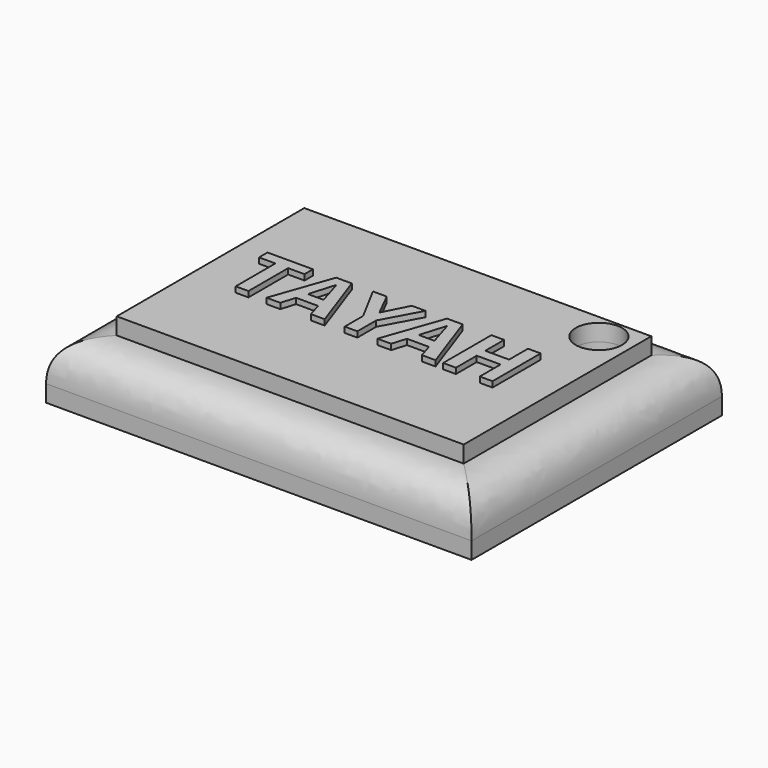
from build123d import *

# Parameters (mm, degrees)
F0_W         = 75.8890584111
F0_H         = 55.81606552
F1_DEPTH     = 10
F2_T1_DEPTH  = 110.8890584111
F2_T3_DEPTH  = 90.81606552
F3_DEPTH     = 3
F4_TEXT_SIZE = 15.0474936518
F6_DEPTH     = 1
F5_R         = 4.1296753225
F7_DEPTH     = 29.6


# Not quite as in the source:
# - a fillet or chamfer that OpenCascade refuses, or shapes differently, is made with other operations: its cross-section is extruded or revolved along the edge and cut away or added
# - Text() gives the source's letters only with a copy of the font that has no kerning and outlines rounded to 1/6400 em; it was checked with that copy


with BuildPart() as f1:
    # F0 (on Top) → F1 (new body)
    with BuildSketch(Plane.XY):
        with Locations((-37.9445292056, 27.90803276)):
            Rectangle(F0_W, F0_H)
    extrude(amount=F1_DEPTH)

    # F2: fillet of radius 7 on 4 edges, made by hand

    # F2_s2 → F2_t1 (cut)
    with BuildSketch(Plane.YZ.offset(-93.3890584111)):
        with BuildLine():
            add(Edge.make_bspline(
                [(0, 3), (0, 10), (7, 10)],
                knots=[0, 0, 0, 1, 1, 1], degree=2, weights=[1, 1, 1]))
            Line((7, 10), (0, 10))
            Line((0, 10), (0, 3))
        make_face()
        with BuildLine():
            add(Edge.make_bspline(
                [(55.81606552, 3), (55.81606552, 10), (48.81606552, 10)],
                knots=[0, 0, 0, 1, 1, 1], degree=2, weights=[1, 1, 1]))
            Line((48.81606552, 10), (55.81606552, 10))
            Line((55.81606552, 10), (55.81606552, 3))
        make_face()
    extrude(amount=F2_T1_DEPTH, mode=Mode.SUBTRACT)

    # F2_s4 → F2_t3 (cut)
    with BuildSketch(Plane.XZ.offset(-73.31606552)):
        with BuildLine():
            add(Edge.make_bspline(
                [(0, 3), (0, 10), (-7, 10)],
                knots=[0, 0, 0, 1, 1, 1], degree=2, weights=[1, 1, 1]))
            Line((-7, 10), (0, 10))
            Line((0, 10), (0, 3))
        make_face()
        with BuildLine():
            add(Edge.make_bspline(
                [(-75.8890584111, 3), (-75.8890584111, 10), (-68.8890584111, 10)],
                knots=[0, 0, 0, 1, 1, 1], degree=2, weights=[1, 1, 1]))
            Line((-68.8890584111, 10), (-75.8890584111, 10))
            Line((-75.8890584111, 10), (-75.8890584111, 3))
        make_face()
    extrude(amount=F2_T3_DEPTH, mode=Mode.SUBTRACT)


with BuildPart() as f3:
    # F3 (new): a face of the model
    f3_faces = [f1.part.faces().sort_by_distance(p)[0] for p in [
        (-37.9445292055, 27.90803276, 10),
    ]]
    extrude(f3_faces, amount=F3_DEPTH)

    # F4 (on face) → F6 (join)
    with BuildSketch(Plane.XY.offset(13)):
        with Locations((-63.6217082658, 22.9155987137)):
            Text('TAYAH', F4_TEXT_SIZE, font='Open Sans', font_style=FontStyle.BOLD, text_align=(TextAlign.LEFT, TextAlign.BOTTOM))
    extrude(amount=F6_DEPTH)


with BuildPart() as f7_tool:
    # F5 (on face) → F7 (new body)
    with BuildSketch(Plane.XY.offset(13)):
        with Locations((-12.6543706283, 44.2115217447)):
            Circle(F5_R)
    extrude(amount=-F7_DEPTH)


with BuildPart() as f1_1:
    add(f1.part)

    # F7: cut by f7_tool
    add(f7_tool.part, mode=Mode.SUBTRACT)


with BuildPart() as f3_1:
    add(f3.part)

    # F7: cut by f7_tool
    add(f7_tool.part, mode=Mode.SUBTRACT)


solid = Compound([f1_1.part, f3_1.part])
